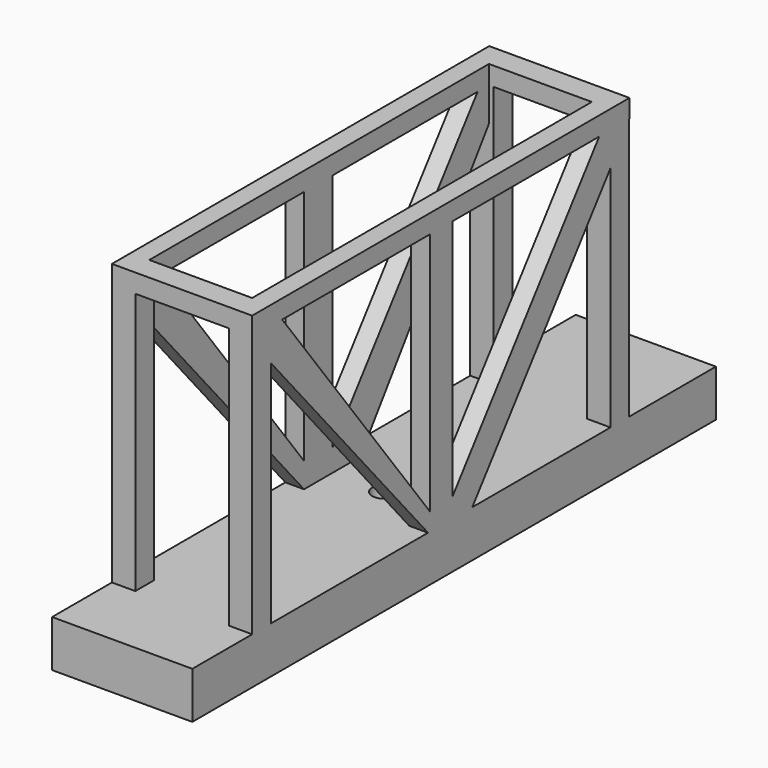
from build123d import *

# Parameters (mm, degrees)
F0_W      = 127
F0_H      = 12.7
F0_W_2    = 25.4
F1_DEPTH  = 38.1
F2_W      = 6.35
F2_H      = 6.35
F3_DEPTH  = 76.2
F4_W      = 6.35
F4_H      = 14.1849974977
F4_H_2    = 13.9073220724
F5_DEPTH  = 5.08
F7_DEPTH  = 5.08
F9_DEPTH  = 119.634
F10_W     = 31.75
F10_H     = 6.35
F11_DEPTH = 5.08
F12_W     = 38.1
F12_H     = 6.4396932721
F13_DEPTH = 5.08
F14_W     = 5.08
F14_H     = 128.0755363405
F15_DEPTH = 5.08
F16_W     = 5.08
F16_H     = 128.120649606
F17_DEPTH = 5.08
F18_W     = 7.6489634812
F18_H     = 71.12
F19_DEPTH = 5.08
F20_W     = 9.6254386008
F20_H     = 73.2569846961
F21_DEPTH = 5.08


# Not quite as in the source:
# - a feature names something its author has since deleted; it is built from what else it names


with BuildPart() as f1:
    # F0 (on Right) → F1 (new body)
    with BuildSketch(Plane.YZ):
        with Locations((-23.7084774733, -8.1166389743)):
            Rectangle(F0_W, F0_H)
        with Locations((-99.9084774733, -8.1166389743)):
            Rectangle(F0_W_2, F0_H)
        with Locations((52.4915225267, -8.1166389743)):
            Rectangle(F0_W_2, F0_H)
    extrude(amount=F1_DEPTH)

    # F2 (on face) → F3 (join)
    with BuildSketch(Plane.XY.offset(-1.7666389743)):
        with Locations((3.175, 32.5670524418)):
            Rectangle(F2_W, F2_H)
        with Locations((34.925, 32.5670524418)):
            Rectangle(F2_W, F2_H)
        with Locations((3.175, -89.113903892)):
            Rectangle(F2_W, F2_H)
        with Locations((34.925, -89.113903892)):
            Rectangle(F2_W, F2_H)
    extrude(amount=F3_DEPTH)

    # F4 (on face) → F5 (join)
    with BuildSketch(Plane.YZ.offset(38.1)):
        with Locations((32.5670524418, 67.3408622769)):
            Rectangle(F4_W, F4_H)
        with Locations((-89.113903892, 67.4796999895)):
            Rectangle(F4_W, F4_H_2)
        Polygon((29.3920524418, 60.2483635281), (29.3920524418, 74.4333610257), (-28.2734257251, -1.7666389743), (-17.538718855, -1.7666389743), align=None)
        Polygon((-32.572824508, -1.7666389743), (-28.2734257251, -1.7666389743), (-85.938903892, 74.4333610257), (-85.938903892, 60.5260389533), align=None)
    extrude(amount=-F5_DEPTH)

    # F6 (on face) → F7 (join)
    with BuildSketch(Plane(origin=(0, 0, 0), x_dir=(0, -1, 0), z_dir=(-1, 0, 0))):
        Polygon((92.288903892, 59.4646334648), (92.288903892, 74.4333610257), (85.938903892, 74.4333610257), (28.2734257251, -1.7666389743), (33.4044694901, -1.7666389743), (85.938903892, 59.4646334648), align=None)
        Polygon((14.3624190241, -1.7666389743), (28.2734257251, -1.7666389743), (-29.3920524418, 74.4333610257), (-35.7420524418, 74.4333610257), (-35.7420524418, 60.1327754557), (-29.3920524418, 60.1327754557), align=None)
    extrude(amount=-F7_DEPTH)

    # F8 (on face) → F9 (cut)
    with BuildSketch(Plane.XY.offset(-1.7666389743)):
        with BuildLine():
            ThreePointArc((19.05, -20.5334774733), (16.8049359697, -25.9535415035), (22.225, -23.7084774733))
            ThreePointArc((22.225, -23.7084774733), (21.2950640303, -21.463413443), (19.05, -20.5334774733))
        make_face()
    extrude(amount=-F9_DEPTH, mode=Mode.SUBTRACT)

    # F10 (on face) → F11 (join)
    with BuildSketch(Plane.XY.offset(74.4333610257)):
        with Locations((15.875, -89.113903892)):
            Rectangle(F10_W, F10_H)
    extrude(amount=-F11_DEPTH)

    # F12 (on face) → F13 (join)
    with BuildSketch(Plane.XY.offset(74.4333610257)):
        with Locations((19.05, 32.6118990779)):
            Rectangle(F12_W, F12_H)
    extrude(amount=-F13_DEPTH)

    # F14 (on face) → F15 (join)
    with BuildSketch(Plane.XY.offset(74.4333610257)):
        with Locations((2.54, -28.2060224563)):
            Rectangle(F14_W, F14_H)
    extrude(amount=-F15_DEPTH)

    # F16 (on face) → F17 (join)
    with BuildSketch(Plane.XY.offset(74.4333610257)):
        with Locations((35.56, -28.228579089)):
            Rectangle(F16_W, F16_H)
    extrude(amount=-F17_DEPTH)

    # F18 (on face) → F19 (join)
    with BuildSketch(Plane.YZ.offset(38.1)):
        with Locations((-28.123093769, 33.7933610257)):
            Rectangle(F18_W, F18_H)
    extrude(amount=-F19_DEPTH)

    # F20 (on face) → F21 (join)
    with BuildSketch(Plane(origin=(0, 0, 0), x_dir=(0, -1, 0), z_dir=(-1, 0, 0))):
        with Locations((28.5917501897, 32.7248686777)):
            Rectangle(F20_W, F20_H)
    extrude(amount=-F21_DEPTH)


solid = f1.part
